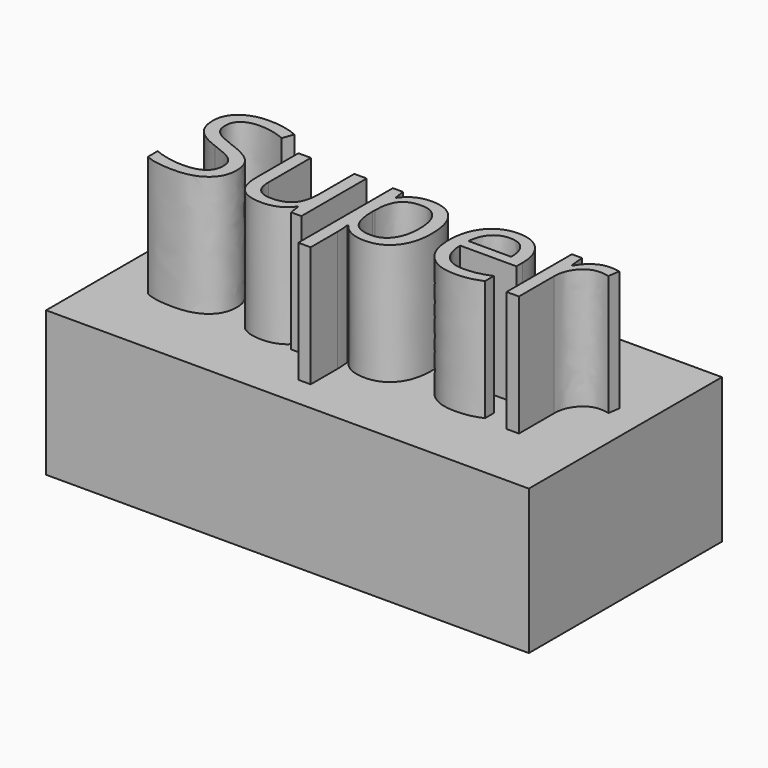
from build123d import *

# Parameters (mm, degrees)
F0_W         = 100
F0_H         = 50
F1_DEPTH     = 30
F2_TEXT_SIZE = 31.5847392711
F3_DEPTH     = 25


# Not quite as in the source:
# - Text() gives the source's letters only with a copy of the font that has no kerning and outlines rounded to 1/6400 em; it was checked with that copy


with BuildPart() as f1:
    # F0 (on Top) → F1 (new body)
    with BuildSketch(Plane.XY):
        Rectangle(F0_W, F0_H)
    extrude(amount=F1_DEPTH)

    # F2 (on face) → F3 (join)
    with BuildSketch(Plane.XY.offset(30)):
        with Locations((-42.3672385514, -10.9424833208)):
            Text('Super', F2_TEXT_SIZE, font='Open Sans', text_align=(TextAlign.LEFT, TextAlign.BOTTOM))
    extrude(amount=F3_DEPTH)


solid = f1.part
